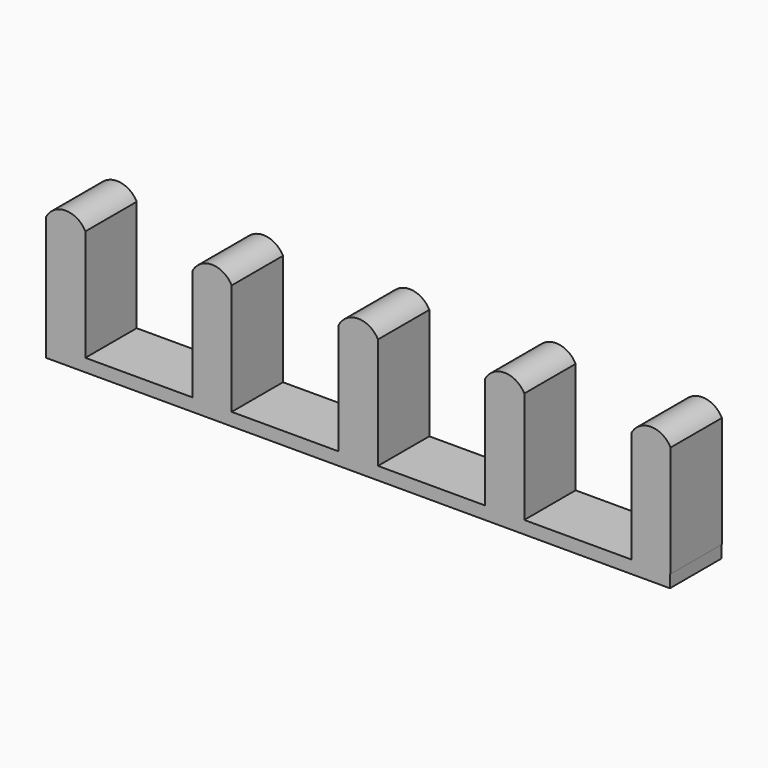
from build123d import *

# Parameters (mm, degrees)
F1_DEPTH = 25


# Not quite as in the source:
# - a feature names something its author has since deleted; it is built from what else it names


with BuildPart() as f1:
    # F0 (on Front) → F1 (new body)
    with BuildSketch(Plane.XZ):
        with BuildLine():
            Line((-57.1667980403, 43.3679167181), (-57.1667980403, 0))
            Line((-57.1667980403, 0), (-41.8604705483, 0))
            Line((-41.8604705483, 0), (-41.8604705483, 43.3679167181))
            ThreePointArc((-41.8604705483, 43.3679167181), (-49.5136342943, 48.0061937124), (-57.1667980403, 43.3679167181))
        make_face()
        with BuildLine():
            Line((-0.1667980403, 43.3679167181), (-0.1667980403, 0))
            Line((-0.1667980403, 0), (15.1395294517, 0))
            Line((15.1395294517, 0), (15.1395294517, 43.3679167181))
            ThreePointArc((15.1395294517, 43.3679167181), (7.4863657057, 48.0061937124), (-0.1667980403, 43.3679167181))
        make_face()
        with BuildLine():
            Line((56.8332019597, 43.3679167181), (56.8332019597, 0))
            Line((56.8332019597, 0), (72.1395294517, 0))
            Line((72.1395294517, 0), (72.1395294517, 43.3679167181))
            ThreePointArc((72.1395294517, 43.3679167181), (64.4863657057, 48.0061937124), (56.8332019597, 43.3679167181))
        make_face()
        with BuildLine():
            Line((113.8332019597, 0), (129.1395294517, 0))
            Line((129.1395294517, 0), (129.1395294517, 43.3679167181))
            ThreePointArc((129.1395294517, 43.3679167181), (121.4863657057, 48.0061937124), (113.8332019597, 43.3679167181))
            Line((113.8332019597, 43.3679167181), (113.8332019597, 0))
        make_face()
        with BuildLine():
            Line((170.8332019597, 0), (185.8886182308, 0))
            Line((185.8886182308, 0), (186.1395294517, 0))
            Line((186.1395294517, 0), (186.1395294517, 43.3679167181))
            ThreePointArc((186.1395294517, 43.3679167181), (178.4863657057, 48.0061937124), (170.8332019597, 43.3679167181))
            Line((170.8332019597, 43.3679167181), (170.8332019597, 0))
        make_face()
        Polygon((-41.8604705483, 0), (-57.1667980403, 0), (-57.1667980403, -4.9899439327), (185.8886182308, -4.9899439327), (185.8886182308, 0), (170.8332019597, 0), (162.9481277168, 0), (140.3730809391, 0), (129.1395294517, 0), (113.8332019597, 0), (105.9481277168, 0), (83.3730809391, 0), (72.1395294517, 0), (56.8332019597, 0), (48.9481277168, 0), (15.1395294517, 0), (-0.1667980403, 0), (-8.0518722832, 0), align=None)
    extrude(amount=F1_DEPTH)


solid = f1.part
